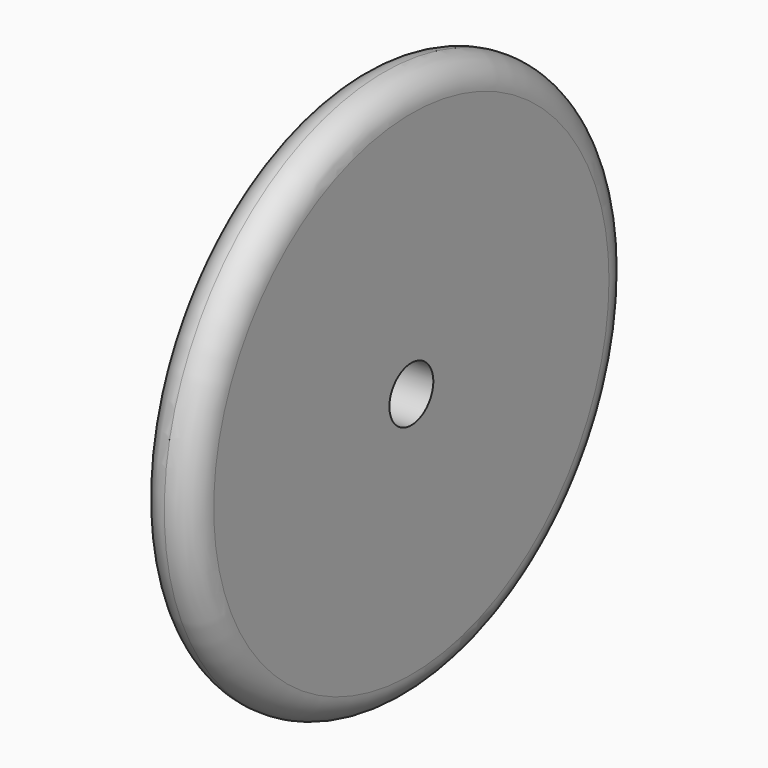
from build123d import *

# Parameters (mm, degrees)
F0_R     = 10
F1_DEPTH = 2
F2_R     = 0.99999
F4_D     = 2


# Not quite as in the source:
# - a fillet or chamfer is up to 0.001 mm smaller than in the source, because OpenCascade refuses the exact size


with BuildPart() as f1:
    # F0 (on Right) → F1 (new body)
    with BuildSketch(Plane.YZ):
        Circle(F0_R)
    extrude(amount=F1_DEPTH)

    # F2 (radius 1 in the source; OpenCascade refuses exactly that, so slightly less here)
    f2_edges = [f1.edges().sort_by_distance(p)[0] for p in [
        (1, 10, 0),
        (0, -10, 0),
        (2, -10, 0),
    ]]
    fillet(f2_edges, radius=F2_R)

    # F4 (through all)
    with Locations(Plane.YZ.offset(2)):
        with Locations((0, 0)):
            Hole(F4_D / 2)


solid = f1.part
